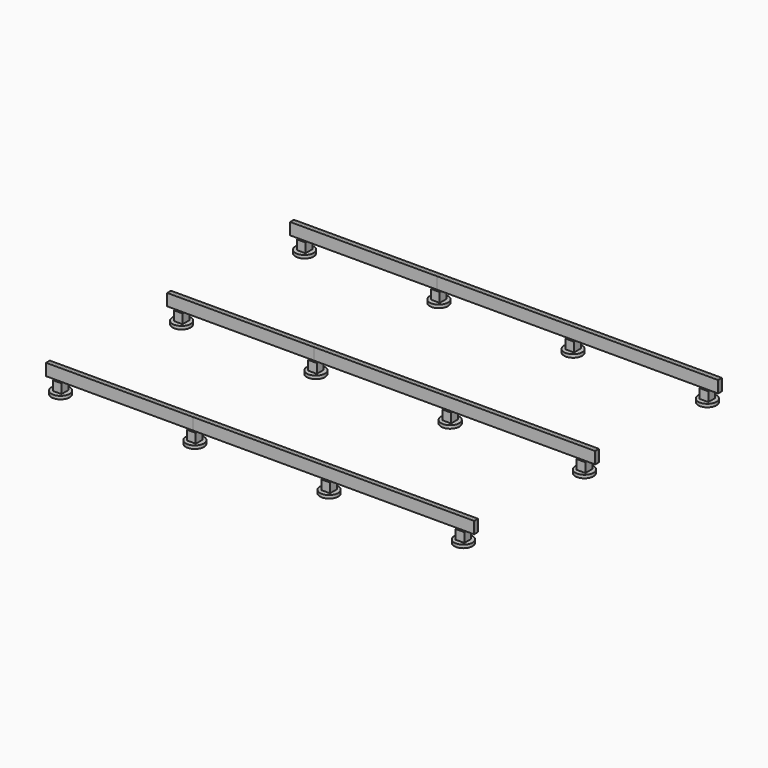
from build123d import *

# Parameters (mm, degrees)
F0_R      = 146.05
F1_DEPTH  = 50.8
F2_W      = 139.7
F2_H      = 139.7
F3_DEPTH  = 152.4
F4_W      = 2367.026
F4_H      = 38.1
F5_DEPTH  = 190.5
F6_W      = 4257.802
F6_H      = 38.1
F6_W_2    = 139.7
F6_W_3    = 133.35
F7_DEPTH  = 190.5
F8_W      = 139.7
F8_H      = 38.1
F8_W_2    = 133.35
F8_W_3    = 4258.02044
F9_DEPTH  = 190.5
F10_W     = 69.85
F10_H     = 38.1
F10_W_2   = 2297.17854
F11_DEPTH = 190.5
F12_W     = 69.85
F12_H     = 38.1
F12_W_2   = 4461.22044
F13_DEPTH = 190.5
F14_W     = 133.35
F14_H     = 38.1
F14_W_2   = 139.7
F14_W_3   = 4258.02044
F15_DEPTH = 190.5
F16_W     = 133.35
F16_H     = 38.1
F16_W_2   = 139.7
F16_W_3   = 2093.97854
F17_DEPTH = 190.5
F18_W     = 133.35
F18_H     = 38.1
F18_W_2   = 139.7
F18_W_3   = 2093.97854
F19_DEPTH = 190.5
F20_W     = 69.84746
F20_H     = 38.1
F20_W_2   = 4461.22298
F21_DEPTH = 190.5
F22_W     = 4461.22298
F22_H     = 38.1
F22_W_2   = 69.84746
F23_DEPTH = 190.5
F24_W     = 2297.39698
F24_H     = 38.1
F24_W_2   = 69.63156
F25_DEPTH = 190.5
F26_W     = 2297.39698
F26_H     = 38.1
F26_W_2   = 69.63156
F27_DEPTH = 190.5


with BuildPart() as f1:
    # F0 (on Top) → F1 (new body)
    with BuildSketch(Plane.XY):
        with Locations((6491.478, 0)):
            Circle(F0_R)
    extrude(amount=F1_DEPTH)


with BuildPart() as f1b:
    # F0 (on Top) → F1, piece 2 (new body)
    with BuildSketch(Plane.XY):
        with Locations((6491.478, -4914.9)):
            Circle(F0_R)
    extrude(amount=F1_DEPTH)


with BuildPart() as f1c:
    # F0 (on Top) → F1, piece 3 (new body)
    with BuildSketch(Plane.XY):
        with Locations((2163.826, -2476.5)):
            Circle(F0_R)
    extrude(amount=F1_DEPTH)


with BuildPart() as f1d:
    # F0 (on Top) → F1, piece 4 (new body)
    with BuildSketch(Plane.XY):
        with Locations((2163.826, -4914.9)):
            Circle(F0_R)
    extrude(amount=F1_DEPTH)


with BuildPart() as f1e:
    # F0 (on Top) → F1, piece 5 (new body)
    with BuildSketch(Plane.XY):
        with Locations((0, -2476.5)):
            Circle(F0_R)
    extrude(amount=F1_DEPTH)


with BuildPart() as f1f:
    # F0 (on Top) → F1, piece 6 (new body)
    with BuildSketch(Plane.XY):
        with Locations((2163.826, 0)):
            Circle(F0_R)
    extrude(amount=F1_DEPTH)


with BuildPart() as f1g:
    # F0 (on Top) → F1, piece 7 (new body)
    with BuildSketch(Plane.XY):
        with Locations((4327.652, -4914.9)):
            Circle(F0_R)
    extrude(amount=F1_DEPTH)


with BuildPart() as f1h:
    # F0 (on Top) → F1, piece 8 (new body)
    with BuildSketch(Plane.XY):
        Circle(F0_R)
    extrude(amount=F1_DEPTH)


with BuildPart() as f1i:
    # F0 (on Top) → F1, piece 9 (new body)
    with BuildSketch(Plane.XY):
        with Locations((4327.652, 0)):
            Circle(F0_R)
    extrude(amount=F1_DEPTH)


with BuildPart() as f1j:
    # F0 (on Top) → F1, piece 10 (new body)
    with BuildSketch(Plane.XY):
        with Locations((4327.652, -2476.5)):
            Circle(F0_R)
    extrude(amount=F1_DEPTH)


with BuildPart() as f1k:
    # F0 (on Top) → F1, piece 11 (new body)
    with BuildSketch(Plane.XY):
        with Locations((6491.478, -2476.5)):
            Circle(F0_R)
    extrude(amount=F1_DEPTH)


with BuildPart() as f1l:
    # F0 (on Top) → F1, piece 12 (new body)
    with BuildSketch(Plane.XY):
        with Locations((0, -4914.9)):
            Circle(F0_R)
    extrude(amount=F1_DEPTH)


with BuildPart() as f3:
    # F2 (on face) → F3 (new body)
    with BuildSketch(Plane.XY.offset(50.8)):
        Rectangle(F2_W, F2_H)
    extrude(amount=F3_DEPTH)


with BuildPart() as f3b:
    # F2 (on face) → F3, piece 2 (new body)
    with BuildSketch(Plane.XY.offset(50.8)):
        with Locations((2163.826, 0)):
            Rectangle(F2_W, F2_H)
    extrude(amount=F3_DEPTH)


with BuildPart() as f3c:
    # F2 (on face) → F3, piece 3 (new body)
    with BuildSketch(Plane.XY.offset(50.8)):
        with Locations((4327.652, 0)):
            Rectangle(F2_W, F2_H)
    extrude(amount=F3_DEPTH)


with BuildPart() as f3d:
    # F2 (on face) → F3, piece 4 (new body)
    with BuildSketch(Plane.XY.offset(50.8)):
        with Locations((6491.478, 0)):
            Rectangle(F2_W, F2_H)
    extrude(amount=F3_DEPTH)


with BuildPart() as f3e:
    # F2 (on face) → F3, piece 5 (new body)
    with BuildSketch(Plane.XY.offset(50.8)):
        with Locations((0, -2476.5)):
            Rectangle(F2_W, F2_H)
    extrude(amount=F3_DEPTH)


with BuildPart() as f3f:
    # F2 (on face) → F3, piece 6 (new body)
    with BuildSketch(Plane.XY.offset(50.8)):
        with Locations((2163.826, -2476.5)):
            Rectangle(F2_W, F2_H)
    extrude(amount=F3_DEPTH)


with BuildPart() as f3g:
    # F2 (on face) → F3, piece 7 (new body)
    with BuildSketch(Plane.XY.offset(50.8)):
        with Locations((4327.652, -2476.5)):
            Rectangle(F2_W, F2_H)
    extrude(amount=F3_DEPTH)


with BuildPart() as f3h:
    # F2 (on face) → F3, piece 8 (new body)
    with BuildSketch(Plane.XY.offset(50.8)):
        with Locations((6491.478, -2476.5)):
            Rectangle(F2_W, F2_H)
    extrude(amount=F3_DEPTH)


with BuildPart() as f3i:
    # F2 (on face) → F3, piece 9 (new body)
    with BuildSketch(Plane.XY.offset(50.8)):
        with Locations((0, -4914.9)):
            Rectangle(F2_W, F2_H)
    extrude(amount=F3_DEPTH)


with BuildPart() as f3j:
    # F2 (on face) → F3, piece 10 (new body)
    with BuildSketch(Plane.XY.offset(50.8)):
        with Locations((2163.826, -4914.9)):
            Rectangle(F2_W, F2_H)
    extrude(amount=F3_DEPTH)


with BuildPart() as f3k:
    # F2 (on face) → F3, piece 11 (new body)
    with BuildSketch(Plane.XY.offset(50.8)):
        with Locations((4327.652, -4914.9)):
            Rectangle(F2_W, F2_H)
    extrude(amount=F3_DEPTH)


with BuildPart() as f3l:
    # F2 (on face) → F3, piece 12 (new body)
    with BuildSketch(Plane.XY.offset(50.8)):
        with Locations((6491.478, -4914.9)):
            Rectangle(F2_W, F2_H)
    extrude(amount=F3_DEPTH)


with BuildPart() as f5:
    # F4 (on face) → F5 (new body)
    with BuildSketch(Plane.XY.offset(203.2)):
        with Locations((980.313, -19.05)):
            Rectangle(F4_W, F4_H)
    extrude(amount=F5_DEPTH)


with BuildPart() as f7:
    # F6 (on face) → F7 (new body)
    with BuildSketch(Plane.XY.offset(203.2)):
        with Locations((2198.751, 19.05)):
            Rectangle(F6_W, F6_H)
        with Locations((0, 19.05)):
            Rectangle(F6_W_2, F6_H)
        with Locations((-136.525, 19.05)):
            Rectangle(F6_W_3, F6_H)
    extrude(amount=F7_DEPTH)


with BuildPart() as f9:
    # F8 (on face) → F9 (new body)
    with BuildSketch(Plane.XY.offset(203.2)):
        with Locations((0, -2457.45)):
            Rectangle(F8_W, F8_H)
        with Locations((-136.525, -2457.45)):
            Rectangle(F8_W_2, F8_H)
        with Locations((2198.86022, -2457.45)):
            Rectangle(F8_W_3, F8_H)
    extrude(amount=F9_DEPTH)


with BuildPart() as f11:
    # F10 (on face) → F11 (new body)
    with BuildSketch(Plane.XY.offset(203.2)):
        with Locations((4362.577, 19.05)):
            Rectangle(F10_W, F10_H)
        with Locations((5546.09127, 19.05)):
            Rectangle(F10_W_2, F10_H)
    extrude(amount=F11_DEPTH)


with BuildPart() as f13:
    # F12 (on face) → F13 (new body)
    with BuildSketch(Plane.XY.offset(203.2)):
        with Locations((2198.751, -19.05)):
            Rectangle(F12_W, F12_H)
        with Locations((4464.28622, -19.05)):
            Rectangle(F12_W_2, F12_H)
    extrude(amount=F13_DEPTH)


with BuildPart() as f15:
    # F14 (on face) → F15 (new body)
    with BuildSketch(Plane.XY.offset(203.2)):
        with Locations((-136.525, -4895.85)):
            Rectangle(F14_W, F14_H)
        with Locations((0, -4895.85)):
            Rectangle(F14_W_2, F14_H)
        with Locations((2198.86022, -4895.85)):
            Rectangle(F14_W_3, F14_H)
    extrude(amount=F15_DEPTH)


with BuildPart() as f17:
    # F16 (on face) → F17 (new body)
    with BuildSketch(Plane.XY.offset(203.2)):
        with Locations((-136.525, -2495.55)):
            Rectangle(F16_W, F16_H)
        with Locations((0, -2495.55)):
            Rectangle(F16_W_2, F16_H)
        with Locations((1116.83927, -2495.55)):
            Rectangle(F16_W_3, F16_H)
    extrude(amount=F17_DEPTH)


with BuildPart() as f19:
    # F18 (on face) → F19 (new body)
    with BuildSketch(Plane.XY.offset(203.2)):
        with Locations((-136.525, -4933.95)):
            Rectangle(F18_W, F18_H)
        with Locations((0, -4933.95)):
            Rectangle(F18_W_2, F18_H)
        with Locations((1116.83927, -4933.95)):
            Rectangle(F18_W_3, F18_H)
    extrude(amount=F19_DEPTH)


with BuildPart() as f21:
    # F20 (on face) → F21 (new body)
    with BuildSketch(Plane.XY.offset(203.2)):
        with Locations((2198.75227, -2495.55)):
            Rectangle(F20_W, F20_H)
        with Locations((4464.28749, -2495.55)):
            Rectangle(F20_W_2, F20_H)
    extrude(amount=F21_DEPTH)


with BuildPart() as f23:
    # F22 (on face) → F23 (new body)
    with BuildSketch(Plane.XY.offset(203.2)):
        with Locations((4464.28749, -4933.95)):
            Rectangle(F22_W, F22_H)
        with Locations((2198.75227, -4933.95)):
            Rectangle(F22_W_2, F22_H)
    extrude(amount=F23_DEPTH)


with BuildPart() as f25:
    # F24 (on face) → F25 (new body)
    with BuildSketch(Plane.XY.offset(203.2)):
        with Locations((5546.20049, -2457.45)):
            Rectangle(F24_W, F24_H)
        with Locations((4362.68622, -2457.45)):
            Rectangle(F24_W_2, F24_H)
    extrude(amount=F25_DEPTH)


with BuildPart() as f27:
    # F26 (on face) → F27 (new body)
    with BuildSketch(Plane.XY.offset(203.2)):
        with Locations((5546.20049, -4895.85)):
            Rectangle(F26_W, F26_H)
        with Locations((4362.68622, -4895.85)):
            Rectangle(F26_W_2, F26_H)
    extrude(amount=F27_DEPTH)


solid = Compound([f1.part, f1b.part, f1c.part, f1d.part, f1e.part, f1f.part, f1g.part, f1h.part, f1i.part, f1j.part, f1k.part, f1l.part, f3.part, f3b.part, f3c.part, f3d.part, f3e.part, f3f.part, f3g.part, f3h.part, f3i.part, f3j.part, f3k.part, f3l.part, f5.part, f7.part, f9.part, f11.part, f13.part, f15.part, f17.part, f19.part, f21.part, f23.part, f25.part, f27.part])
